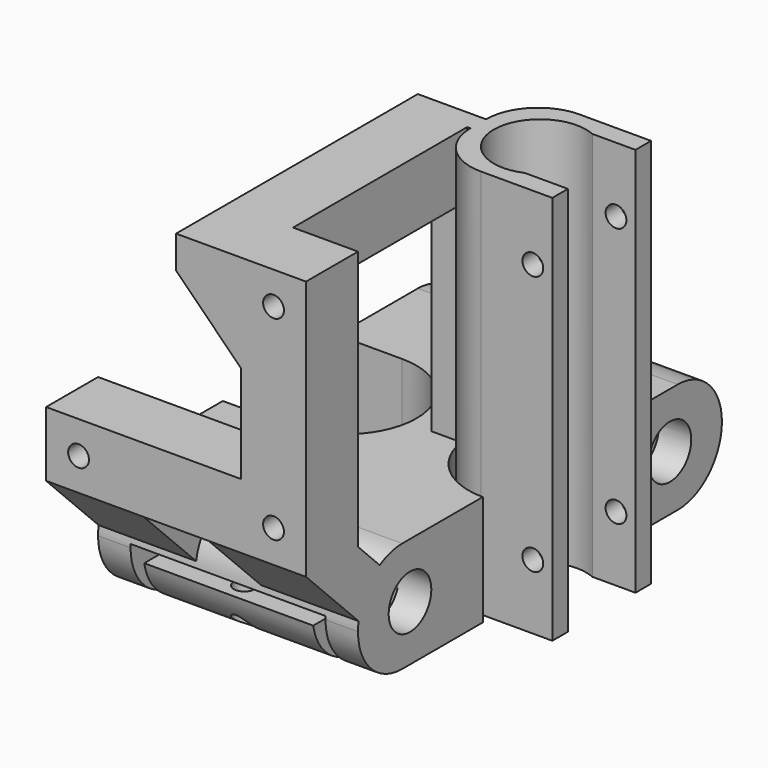
from build123d import *

# Parameters (mm, degrees)
F1_R      = 4.1
F2_DEPTH  = 40
F3_R      = 11
F4_DEPTH  = 17
F5_W      = 6
F5_H      = 3
F6_DEPTH  = 60
F7_R      = 1.6
F8_DEPTH  = 19
F10_DEPTH = 17
F11_W     = 2
F11_H     = 7
F11_H_2   = 2
F11_W_2   = 26
F12_DEPTH = 15
F13_R     = 1.6
F14_DEPTH = 17
F16_DEPTH = 4.5
F19_DEPTH = 15
F21_R     = 1.6
F22_DEPTH = 10
F24_DEPTH = 46.5


# Not quite as in the source:
# - a pattern or mirror of a feature is missing from the dataset's text; its kind, count and spacing are read off the source's solid


with BuildPart() as f2:
    # F1 (on Right) → F2 (new body)
    with BuildSketch(Plane.YZ):
        with BuildLine():
            ThreePointArc((-35, 8.5), (-32.5104076401, 2.4895923599), (-26.5, 0))
            Line((-26.5, 0), (26.5, 0))
            ThreePointArc((26.5, 0), (32.5104076401, 2.4895923599), (35, 8.5))
            ThreePointArc((35, 8.5), (32.5104076401, 14.5104076401), (26.5, 17))
            Line((26.5, 17), (-26.5, 17))
            ThreePointArc((-26.5, 17), (-32.5104076401, 14.5104076401), (-35, 8.5))
        make_face()
        with Locations((-25, 8.5)):
            Circle(F1_R, mode=Mode.SUBTRACT)
        with Locations((25, 8.5)):
            Circle(F1_R, mode=Mode.SUBTRACT)
    extrude(amount=-F2_DEPTH)

    # F3 (on Top) → F4 (cut)
    with BuildSketch(Plane.XY):
        Circle(F3_R)
    extrude(amount=F4_DEPTH, mode=Mode.SUBTRACT)

    # F5 (on Top) → F6 (join)
    with BuildSketch(Plane.XY):
        with BuildLine():
            Line((9.5, 6.5), (9.5, 9.5))
            Line((9.5, 9.5), (-1.5, 9.5))
            ThreePointArc((-1.5, 9.5), (-7.1568542495, 7.1568542495), (-9.5, 1.5))
            Line((-9.5, 1.5), (-9.5, -1.5))
            ThreePointArc((-9.5, -1.5), (-7.1568542495, -7.1568542495), (-1.5, -9.5))
            Line((-1.5, -9.5), (9.5, -9.5))
            Line((9.5, -9.5), (9.5, -6.5))
            Line((9.5, -6.5), (2.8565713714, -6.5))
            ThreePointArc((2.8565713714, -6.5), (-7.1, 0), (2.8565713714, 6.5))
            Line((2.8565713714, 6.5), (9.5, 6.5))
        make_face()
        with Locations((-12.5, 0)):
            Rectangle(F5_W, F5_H)
    extrude(amount=F6_DEPTH)

    # F7 (on face) → F8 (cut)
    with BuildSketch(Plane.XZ.offset(9.5)):
        with Locations((6.5, 50)):
            Circle(F7_R)
        with Locations((6.5, 10)):
            Circle(F7_R)
    extrude(amount=-F8_DEPTH, mode=Mode.SUBTRACT)

    # F9 (on Top) → F10 (cut)
    with BuildSketch(Plane.XY):
        with BuildLine():
            ThreePointArc((-19, 0), (-22.2218254069, 7.7781745931), (-30, 11))
            Line((-30, 11), (-41, 11))
            Line((-41, 11), (-41, -11))
            Line((-41, -11), (-30, -11))
            ThreePointArc((-30, -11), (-22.2218254069, -7.7781745931), (-19, 0))
        make_face()
    extrude(amount=F10_DEPTH, mode=Mode.SUBTRACT)

    # F11 (on offset) → F12 (cut)
    with BuildSketch(Plane.XZ.offset(21)):
        with Locations((-6, 3.5)):
            Rectangle(F11_W, F11_H)
        with Locations((-6, 8)):
            Rectangle(F11_W, F11_H_2)
        with Locations((-20, 8)):
            Rectangle(F11_W_2, F11_H_2)
        with Locations((-34, 8)):
            Rectangle(F11_W, F11_H_2)
        with Locations((-34, 3.5)):
            Rectangle(F11_W, F11_H)
    f12 = extrude(amount=F12_DEPTH, mode=Mode.SUBTRACT)

    # F12_copies: F12 across plane
    add(f12.mirror(Plane.ZX), mode=Mode.SUBTRACT)

    # F13 (on Top) → F14 (cut)
    with BuildSketch(Plane.XY):
        with Locations((-20, -31.8666002653)):
            Circle(F13_R)
    f14 = extrude(amount=F14_DEPTH, mode=Mode.SUBTRACT)

    # F14_copies: F14 across plane
    add(f14.mirror(Plane.ZX), mode=Mode.SUBTRACT)

    # F15 (on face) → F16 (cut)
    with BuildSketch(Plane.XY.offset(17)):
        Polygon((-21.6165807537, -29.0666002653), (-23.2331615075, -31.8666002653), (-21.6165807537, -34.6666002653), (-18.3834192463, -34.6666002653), (-16.7668384925, -31.8666002653), (-18.3834192463, -29.0666002653), align=None)
    f16 = extrude(amount=-F16_DEPTH, mode=Mode.SUBTRACT)

    # F16_copies: F16 across plane
    add(f16.mirror(Plane.ZX), mode=Mode.SUBTRACT)

    # F18 (on face) → F19 (join)
    with BuildSketch(Plane(origin=(-40, 0, 0), x_dir=(0, -1, 0), z_dir=(-1, 0, 0))):
        Polygon((34.8862050714, 9.8862050714), (45, 20), (35, 20), (29.8862050714, 14.8862050714), align=None)
    f19 = extrude(amount=-F19_DEPTH)

    # F19_copies: F19 across plane
    add(f19.mirror(Plane(origin=(-20, 0, 0), x_dir=(0, 0, 1), z_dir=(1, 0, 0))))

    # F21 (on offset) → F22 (join)
    with BuildSketch(Plane.XZ.offset(45)):
        Polygon((-40, 20), (0, 20), (0, 60), (-10, 60), (-20, 60), (-20, 55), (-10, 45), (-10, 30), (-40, 30), align=None)
        with Locations((-35, 25)):
            Circle(F21_R, mode=Mode.SUBTRACT)
        with Locations((-5, 25)):
            Circle(F21_R, mode=Mode.SUBTRACT)
        with Locations((-5, 55)):
            Circle(F21_R, mode=Mode.SUBTRACT)
    extrude(amount=-F22_DEPTH)

    # F23 (on face) → F24 (join)
    with BuildSketch(Plane(origin=(0, 1.5, 0), x_dir=(-1, 0, 0), z_dir=(0, 1, 0))):
        Polygon((20, 60), (10, 60), (10, 50), (15, 50), (20, 55), align=None)
    extrude(amount=-F24_DEPTH)


solid = f2.part
